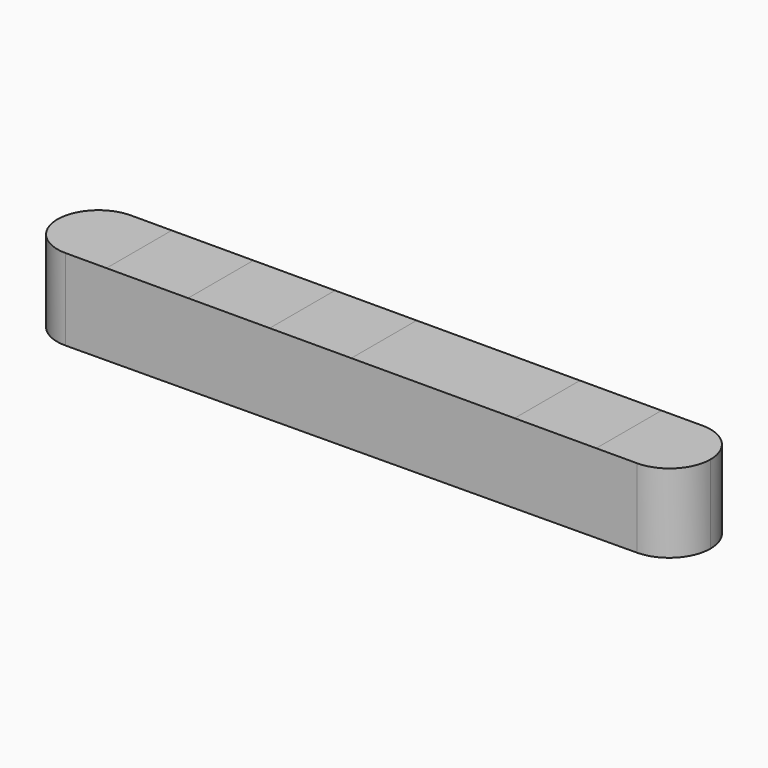
from build123d import *

# Parameters (mm, degrees)
F1_DEPTH = 4
F2_R     = 3.99999


# Not quite as in the source:
# - a fillet or chamfer is up to 0.001 mm smaller than in the source, because OpenCascade refuses the exact size
# - ends of sketch curves that miss each other by under 0.0002 mm in the source are joined
# - a feature names something its author has since deleted; it is built from what else it names


with BuildPart() as f1:
    # F0 (on Front) → F1 (new body, symmetric)
    with BuildSketch(Plane.XZ):
        Polygon((-14.732436277, -7.7009890229), (-14.732436277, 0), (-22.7324279615, -0.0115346295), (-22.721270651, -7.7498318101), align=None)
        Polygon((-22.721270651, -7.7498318101), (-22.7324279615, -0.0115346295), (-30.732419646, -0.0230692591), (-30.7212084456, -7.7987424823), align=None)
        Polygon((-30.7212084456, -7.7987424823), (-30.732419646, -0.0230692591), (-38.7324113305, -0.0346038886), (-38.7211462402, -7.8476531545), align=None)
        Polygon((-38.7211462402, -7.8476531545), (-38.7324113305, -0.0346038886), (-46.732403015, -0.0461385181), (-46.6844078154, -7.8963395926), align=None)
        Polygon((-46.6844078154, -7.8963395926), (-46.732403015, -0.0461385181), (-54.7323946996, -0.0576731477), (-54.7210218294, -7.9454744989), align=None)
        Polygon((-54.7210218294, -7.9454744989), (-54.7323946996, -0.0576731477), (-62.7323863841, -0.0692077772), (-62.7208598391, -7.994384561), align=None)
        Polygon((-62.7208598391, -7.994384561), (-62.7322865984, -0.0692076333), (-70.7323780686, -0.0807424068), (-70.7208974186, -8.0432958433), align=None)
        Polygon((-70.7208974186, -8.0432958433), (-70.7323780686, -0.0807424068), (-78.7323697531, -0.0922770363), (-78.7323697531, -8.0922770363), align=None)
    extrude(amount=F1_DEPTH, both=True)

    # F2 (radius 4 in the source; OpenCascade refuses exactly that, so slightly less here)
    f2_edges = [f1.edges().sort_by_distance(p)[0] for p in [
        (-78.73237, 4, -4.092277),
        (-78.73237, -4, -4.092277),
        (-14.732436, 4, -3.850495),
        (-14.732436, -4, -3.850495),
    ]]
    fillet(f2_edges, radius=F2_R)


solid = f1.part
